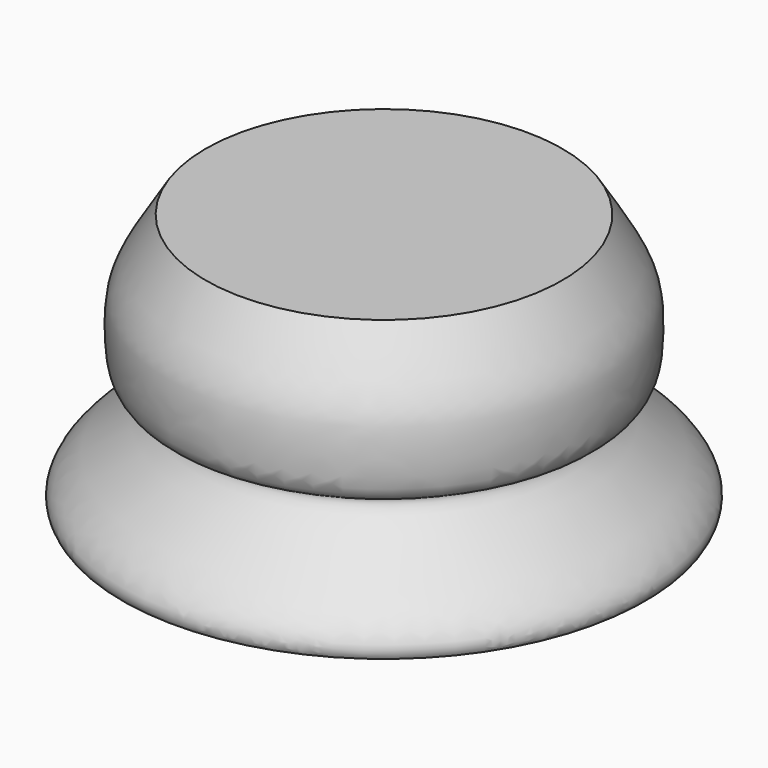
from build123d import *


with BuildPart() as f2:
    # F0 (on Front) → F2 (revolve)
    with BuildSketch(Plane.XZ):
        with BuildLine():
            Line((0, 22.9981895605), (-6.1160139578, 22.9981895605))
            add(Edge.make_bspline(
                [(-6.1160139578, 22.9981895605), (-6.5272548109, 22.3282296666), (-7.4859096846, 20.904050977), (-7.4873686315, 19.7136508406), (-7.4592975783, 17.9435108088), (-5.9023238156, 17.8655136182), (-6.89405113, 16.5827279586), (-9.3976303075, 14.9604288728), (-8.9747941843, 14.2645384553), (-8.9591628024, 14.24242636)],
                knots=[0.4716491127, 0.4716491127, 0.4716491127, 0.4716491127, 0.529700376, 0.5922757431, 0.6536436214, 0.7027449596, 0.7585125505, 0.8480046848, 0.8509865829, 0.8509865829, 0.8509865829, 0.8509865829], degree=3))
            Line((-8.9591628024, 14.24242636), (0, 14.2019145489))
            Line((0, 14.2019145489), (0, 22.9981895605))
        make_face()
    revolve(axis=Axis((0, 0, 28.1776376069), (0, 0, -1)))


solid = f2.part
